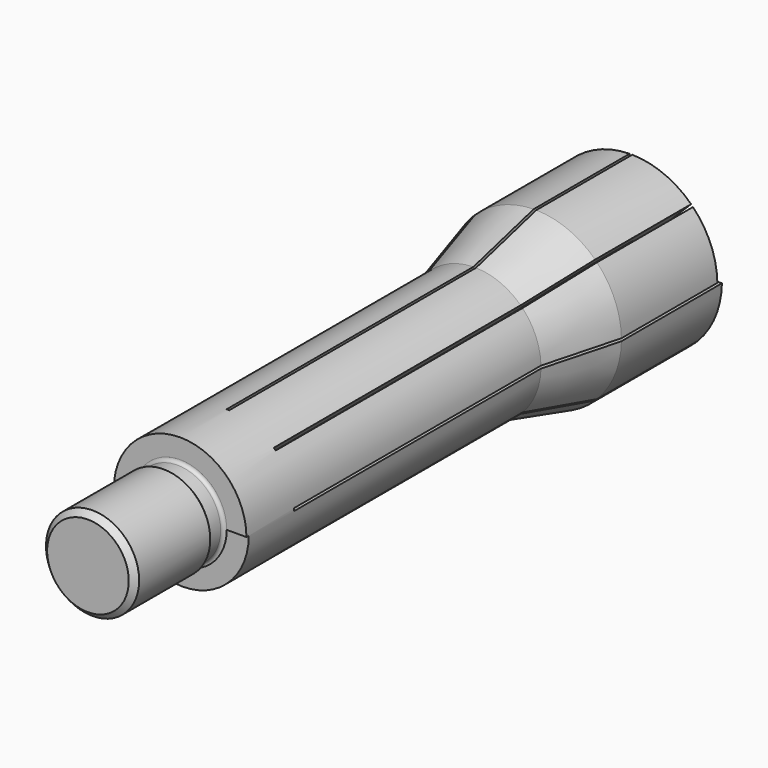
from build123d import *

# Parameters (mm, degrees)
F0_R              = 76.2
F1_DEPTH          = 501.65
F2_R              = 41.0464
F3_DEPTH          = 101.6
F6_SIZE           = 5.08
F11_W             = 1.1684
F11_H             = 449.072
F12_DEPTH         = 104.394
F12_COPIES_COUNT  = 3
F12_COPIES_ANGLE  = 90
F12_COPIES1_COUNT = 2
F12_COPIES1_ANGLE = 45
F12_COPIES2_COUNT = 2
F12_COPIES2_ANGLE = 90
F12_COPIES3_COUNT = 2
F12_COPIES3_PITCH = 93.334588
F15_DEPTH         = 2.54
F17_DEPTH         = 5


# Not quite as in the source:
# - a pattern or mirror of a feature is missing from the dataset's text; its kind, count and spacing are read off the source's solid


with BuildPart() as f1:
    # F0 (on Front) → F1 (new body)
    with BuildSketch(Plane.XZ):
        Circle(F0_R)
    extrude(amount=F1_DEPTH)

    # F2 (on face) → F3 (join)
    with BuildSketch(Plane.XZ.offset(501.65)):
        Circle(F2_R)
    extrude(amount=F3_DEPTH)

    # F4 (on Top) → F5 (revolve, cut)
    with BuildSketch(Plane.XY):
        with BuildLine():
            Line((46.1570850583, -524.9470850583), (47.0411814749, -501.65))
            Line((47.0411814749, -501.65), (41.148, -501.65))
            ThreePointArc((41.148, -501.65), (38.9927385309, -502.5427385309), (38.1, -504.698))
            Line((38.1, -504.698), (38.1, -516.89))
            Line((38.1, -516.89), (46.1570850583, -524.9470850583))
        make_face()
    revolve(axis=Axis((0, -539.7904975197, 0), (0, 1, 0)), mode=Mode.SUBTRACT)

    # F6
    f6_edges = [f1.edges().sort_by_distance(p)[0] for p in [
        (-41.0464, -603.25, 0),
    ]]
    chamfer(f6_edges, length=F6_SIZE)

    # F7 (on Top) → F9 (revolve, cut)
    with BuildSketch(Plane.XY):
        with BuildLine():
            Line((24.8276516795, 11.305465363), (0, 0))
            Line((0, 0), (0, -469.9))
            Line((0, -469.9), (22.225, -469.9))
            ThreePointArc((22.225, -469.9), (31.2052561211, -466.1802561211), (34.925, -457.2))
            Line((34.925, -457.2), (34.925, -178.4670655777))
            Line((34.925, -178.4670655777), (56.134, -99.314))
            Line((56.134, -99.314), (56.134, -51.4132877862))
            Line((56.134, -51.4132877862), (38.354, -41.148))
            Line((38.354, -41.148), (38.354, -16.7454057367))
            Line((38.354, -16.7454057367), (47.1501936142, -2.938147487))
            ThreePointArc((47.1501936142, -2.938147487), (49.4514506124, -0.7827851013), (52.5057292951, 0))
            Line((52.5057292951, 0), (57.8081831336, 10.0514525548))
            Line((57.8081831336, 10.0514525548), (24.8276516795, 11.305465363))
        make_face()
    revolve(axis=Axis((0, 0, 0), (0, 1, 0)), mode=Mode.SUBTRACT)

    # F8 (on Top) → F10 (revolve, cut)
    with BuildSketch(Plane.XY):
        Polygon((122.1472248435, -191.5448755026), (76.2, -110.744), (58.42, -177.0998633586), (58.42, -484.9582612514), (58.42, -521.4050412178), (105.8315560222, -521.4050412178), align=None)
    revolve(axis=Axis((0, 0, 0), (0, 1, 0)), mode=Mode.SUBTRACT)

    # F11 (on Top) → F12 (cut)
    with BuildSketch(Plane.XY):
        with Locations((0.5842, -224.536)):
            Rectangle(F11_W, F11_H)
        with Locations((-0.5842, -224.536)):
            Rectangle(F11_W, F11_H)
    f12 = extrude(amount=F12_DEPTH, mode=Mode.SUBTRACT)

    # F12_copies: F12 ×3 about axis
    f12_copies_axis = Axis((0, 0, 0), (0, -1, 0))
    for i in range(1, F12_COPIES_COUNT):
        add(f12.rotate(f12_copies_axis, i * F12_COPIES_ANGLE / (F12_COPIES_COUNT - 1)), mode=Mode.SUBTRACT)

    # F12_copies1: F12 ×2 about axis
    f12_copies1_axis = Axis((0, 0, 0), (0, 1, 0))
    for i in range(1, F12_COPIES1_COUNT):
        add(f12.rotate(f12_copies1_axis, i * F12_COPIES1_ANGLE / (F12_COPIES1_COUNT - 1)), mode=Mode.SUBTRACT)

    # F12_copies2: F12 ×2 about axis
    f12_copies2_axis = Axis((0, 0, 0), (0, 1, 0))
    for i in range(1, F12_COPIES2_COUNT):
        add(f12.rotate(f12_copies2_axis, i * F12_COPIES2_ANGLE / (F12_COPIES2_COUNT - 1)), mode=Mode.SUBTRACT)

    # F12_copies3: F12 ×2
    with Locations(*[(0, 0, -i * F12_COPIES3_PITCH) for i in range(1, F12_COPIES3_COUNT)]):
        add(f12, mode=Mode.SUBTRACT)

    # F12_copies4: F12 across plane
    add(f12.mirror(Plane(origin=(0, 0, 0), x_dir=(-0.9238795325, 0, -0.3826834324), z_dir=(0.3826834324, 0, -0.9238795325))), mode=Mode.SUBTRACT)

    # F12_copies5: F12 across plane
    add(f12.mirror(Plane(origin=(0, 0, 0), x_dir=(-0.9238795325, 0, 0.3826834324), z_dir=(-0.3826834324, 0, -0.9238795325))), mode=Mode.SUBTRACT)

    # F14 (on offset) → F15 (cut)
    with BuildSketch(Plane.XZ.offset(501.65)):
        Polygon((99.8721420765, -39.6551303566), (84.6954882145, 0), (-85.1850584149, 0), (-16.155783087, -94.9764549732), (63.6440142989, -83.2267925143), align=None)
    extrude(amount=-F15_DEPTH, mode=Mode.SUBTRACT)

    # F16 (on Front) → F17 (cut)
    with BuildSketch(Plane.XZ):
        Polygon((-94.7459638119, 0), (0, 0), (94.7459638119, 0), (94.7459638119, 80.5829763412), (0, 80.5829763412), (-94.7459638119, 80.5829763412), align=None)
    extrude(amount=F17_DEPTH, mode=Mode.SUBTRACT)


solid = f1.part
